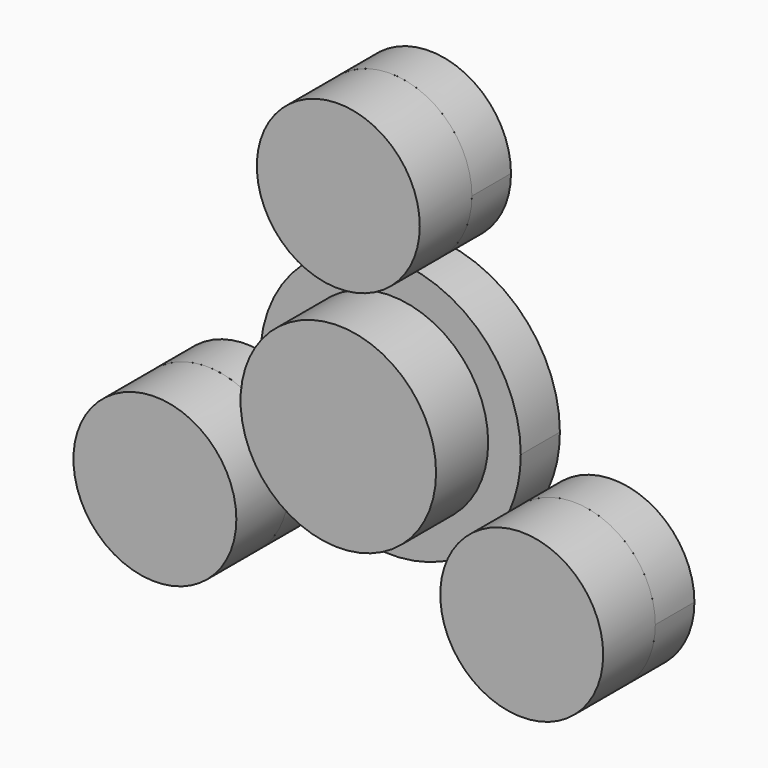
from build123d import *

# Parameters (mm, degrees)
F1_DEPTH = 4.7625
F2_R     = 9.525
F3_DEPTH = 6.35
F2_R_2   = 7.9375


with BuildPart() as f1:
    # F0 (on Front) → F1 (new body)
    with BuildSketch(Plane.XZ):
        with BuildLine():
            ThreePointArc((10.9985225391, -6.3500001541), (12.2672579708, -3.2870019587), (12.7, 0))
            ThreePointArc((12.7, 0), (8.9802561389, 8.9802561032), (5.05e-08, 12.7))
            ThreePointArc((5.05e-08, 12.7), (-10.9985226051, 6.3500000397), (-10.9985226487, -6.3499999643))
            ThreePointArc((-10.9985226487, -6.3499999643), (-1.096e-07, -12.7), (10.9985225391, -6.3500001541))
        make_face()
    extrude(amount=F1_DEPTH)

    # F2 (on face) → F3 (join)
    with BuildSketch(Plane.XZ.offset(4.7625)):
        Circle(F2_R)
    extrude(amount=F3_DEPTH)


with BuildPart() as f1b:
    # F0 (on Front) → F1, piece 2 (new body)
    with BuildSketch(Plane.XZ):
        with BuildLine():
            ThreePointArc((25.8100992706, -10.31875), (19.9269753552, -2.6517137308), (10.9985225391, -6.3500001541))
            ThreePointArc((10.9985225391, -6.3500001541), (15.818223186, -17.9857862692), (25.8100992706, -10.31875))
        make_face()
    extrude(amount=F1_DEPTH)


with BuildPart() as f1c:
    # F0 (on Front) → F1, piece 3 (new body)
    with BuildSketch(Plane.XZ):
        with BuildLine():
            ThreePointArc((-9.9350992706, -10.31875), (-10.2055630298, -8.2643738096), (-10.9985226487, -6.3499999643))
            ThreePointArc((-10.9985226487, -6.3499999643), (-25.5396355114, -12.3731261904), (-9.9350992706, -10.31875))
        make_face()
    extrude(amount=F1_DEPTH)


with BuildPart() as f1d:
    # F0 (on Front) → F1, piece 4 (new body)
    with BuildSketch(Plane.XZ):
        with BuildLine():
            ThreePointArc((7.9375, 20.6375), (-5.6126600935, 26.2501600578), (5.05e-08, 12.7))
            ThreePointArc((5.05e-08, 12.7), (5.6126600935, 15.0248399422), (7.9375, 20.6375))
        make_face()
    extrude(amount=F1_DEPTH)


with BuildPart() as f3:
    # F2 (on face) → F3, piece 2 (new body)
    with BuildSketch(Plane.XZ.offset(4.7625)):
        with Locations((-17.8725992706, -10.31875)):
            Circle(F2_R_2)
    extrude(amount=F3_DEPTH)


with BuildPart() as f3b:
    # F2 (on face) → F3, piece 3 (new body)
    with BuildSketch(Plane.XZ.offset(4.7625)):
        with Locations((0, 20.6375)):
            Circle(F2_R_2)
    extrude(amount=F3_DEPTH)


with BuildPart() as f3c:
    # F2 (on face) → F3, piece 4 (new body)
    with BuildSketch(Plane.XZ.offset(4.7625)):
        with Locations((17.8725992706, -10.31875)):
            Circle(F2_R_2)
    extrude(amount=F3_DEPTH)


solid = Compound([f1.part, f1b.part, f1c.part, f1d.part, f3.part, f3b.part, f3c.part])
